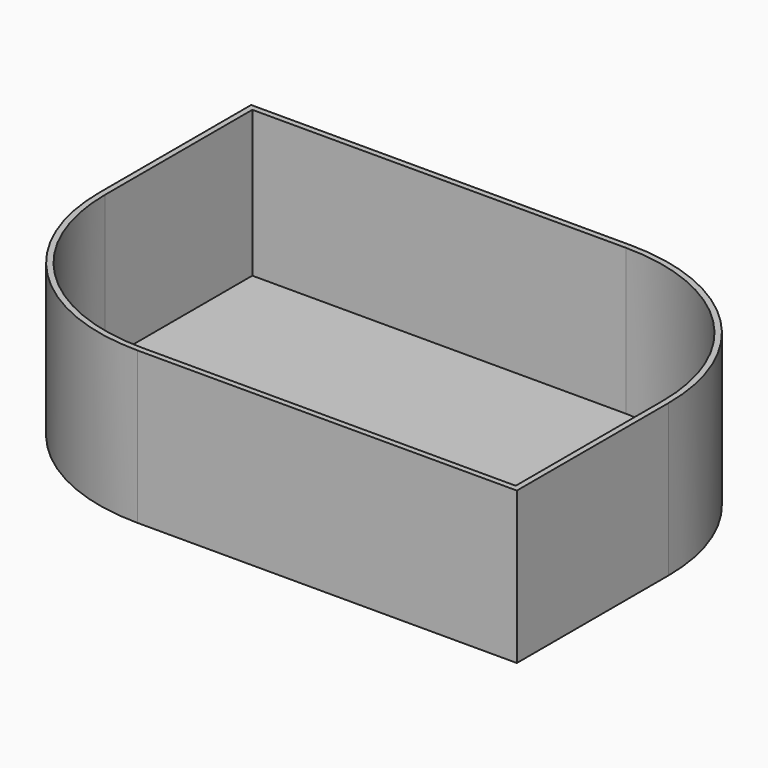
from build123d import *

# Parameters (mm, degrees)
F1_DEPTH = 4000
F2_T     = -152.4


# Not quite as in the source:
# - the program builds the solid bodies; features that only make, move or delete a surface that nothing else refers to are left out


with BuildPart() as f1:
    # F0 (on Top) → F1 (new body)
    with BuildSketch(Plane.XY):
        with BuildLine():
            Line((-1945.6784874201, 4850.0422537327), (-11945.6784874201, 4850.0422537327))
            Line((-11945.6784874201, 4850.0422537327), (-11945.6784874201, -149.9577462673))
            ThreePointArc((-11945.6784874201, -149.9577462673), (-10481.2123933528, -3685.4916522001), (-6945.6784874201, -5149.9577462673))
            Line((-6945.6784874201, -5149.9577462673), (3054.3215125799, -5149.9577462673))
            Line((3054.3215125799, -5149.9577462673), (3054.3215125799, -149.9577462673))
            ThreePointArc((3054.3215125799, -149.9577462673), (1589.8554185127, 3385.5761596654), (-1945.6784874201, 4850.0422537327))
        make_face()
    extrude(amount=F1_DEPTH)

    # F2
    f2_openings = [f1.faces().sort_by_distance(p)[0] for p in [
        (-4445.678487, -149.957746, 4000),
    ]]
    offset(amount=F2_T, openings=f2_openings)


solid = f1.part
